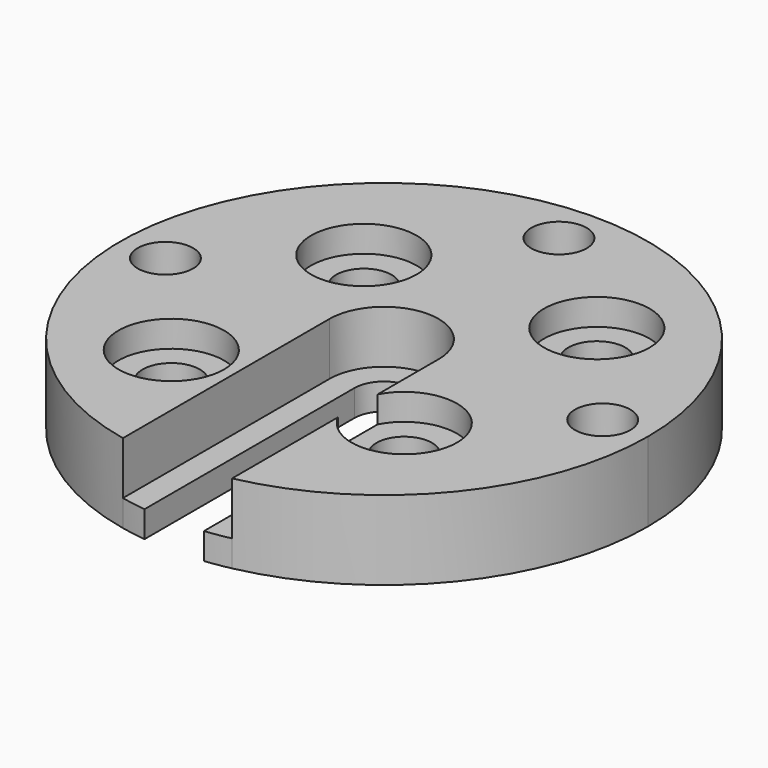
from build123d import *

# Parameters (mm, degrees)
F1_DEPTH = 1.5
F0_R     = 3
F0_R_2   = 1.575
F2_DEPTH = 4.5
F0_R_3   = 1.625
F3_DEPTH = 3


# Not quite as in the source:
# - a feature names something its author has since deleted; it is built from what else it names


with BuildPart() as f1:
    # F0 (on Top) → F1 (new body)
    with BuildSketch(Plane.XY):
        with BuildLine():
            Line((-1.685, -4.7075232341), (-1.685, -2.6020712903))
            ThreePointArc((-1.685, -2.6020712903), (-2.7233710728, -1.4809625248), (-3.1, 0))
            Line((-3.1, 0), (-3.1, -3.9230090492))
            ThreePointArc((-3.1, -3.9230090492), (-2.4244425909, -4.3728798432), (-1.685, -4.7075232341))
        make_face()
        with BuildLine():
            Line((-1.685, -14.905058705), (-1.685, -4.7075232341))
            ThreePointArc((-1.685, -4.7075232341), (-2.4244425909, -4.3728798432), (-3.1, -3.9230090492))
            Line((-3.1, -3.9230090492), (-3.1, -14.6761711628))
            ThreePointArc((-3.1, -14.6761711628), (-2.3952356099, -14.8075266798), (-1.685, -14.905058705))
        make_face()
        with BuildLine():
            ThreePointArc((3.1, -3.9230090492), (2.4244425909, -4.3728798432), (1.685, -4.7075232341))
            Line((1.685, -4.7075232341), (1.685, -14.905058705))
            ThreePointArc((1.685, -14.905058705), (2.3952356099, -14.8075266798), (3.1, -14.6761711628))
            Line((3.1, -14.6761711628), (3.1, -7.1604074647))
            ThreePointArc((3.1, -7.1604074647), (2.7452425971, -5.7452425971), (3.1, -4.3300777296))
            Line((3.1, -4.3300777296), (3.1, -3.9230090492))
        make_face()
        with BuildLine():
            ThreePointArc((-1.685, 0), (0, 1.685), (1.685, 0))
            Line((1.685, 0), (1.685, -2.6020712903))
            ThreePointArc((1.685, -2.6020712903), (2.7233710728, -1.4809625248), (3.1, 0))
            ThreePointArc((3.1, 0), (0, 3.1), (-3.1, 0))
            ThreePointArc((-3.1, 0), (-2.7233710728, -1.4809625248), (-1.685, -2.6020712903))
            Line((-1.685, -2.6020712903), (-1.685, 0))
        make_face()
        with BuildLine():
            ThreePointArc((-3.1, 0), (0, 3.1), (3.1, 0))
            Line((3.1, 0), (3.1, -3.9230090492))
            ThreePointArc((3.1, -3.9230090492), (4.5, -2.1794494718), (5, 0))
            ThreePointArc((5, 0), (-2.1794494718, 4.5), (-3.1, -3.9230090492))
            Line((-3.1, -3.9230090492), (-3.1, 0))
        make_face()
        with BuildLine():
            ThreePointArc((3.1, 0), (2.7233710728, -1.4809625248), (1.685, -2.6020712903))
            Line((1.685, -2.6020712903), (1.685, -4.7075232341))
            ThreePointArc((1.685, -4.7075232341), (2.4244425909, -4.3728798432), (3.1, -3.9230090492))
            Line((3.1, -3.9230090492), (3.1, 0))
        make_face()
        with BuildLine():
            Line((3.1, -7.1604074647), (3.1, -4.3300777296))
            ThreePointArc((3.1, -4.3300777296), (2.7452425971, -5.7452425971), (3.1, -7.1604074647))
        make_face()
    extrude(amount=F1_DEPTH)

    # F0 (on Top) → F2 (join)
    with BuildSketch(Plane.XY):
        with BuildLine():
            ThreePointArc((-3.1, 0), (0, 3.1), (3.1, 0))
            Line((3.1, 0), (3.1, -3.9230090492))
            ThreePointArc((3.1, -3.9230090492), (4.5, -2.1794494718), (5, 0))
            ThreePointArc((5, 0), (-2.1794494718, 4.5), (-3.1, -3.9230090492))
            Line((-3.1, -3.9230090492), (-3.1, 0))
        make_face()
        with BuildLine():
            ThreePointArc((5, 0), (4.5, -2.1794494718), (3.1, -3.9230090492))
            Line((3.1, -3.9230090492), (3.1, -4.3300777296))
            ThreePointArc((3.1, -4.3300777296), (6.4747191933, -2.8352831652), (8.7452425971, -5.7452425971))
            ThreePointArc((8.7452425971, -5.7452425971), (6.4747191933, -8.6552020291), (3.1, -7.1604074647))
            Line((3.1, -7.1604074647), (3.1, -14.6761711628))
            ThreePointArc((3.1, -14.6761711628), (11.6511801977, -9.4472218138), (15, 0))
            ThreePointArc((15, 0), (-9.4472218138, 11.6511801977), (-3.1, -14.6761711628))
            Line((-3.1, -14.6761711628), (-3.1, -3.9230090492))
            ThreePointArc((-3.1, -3.9230090492), (-2.1794494718, 4.5), (5, 0))
        make_face()
        with Locations((-6.7175144213, -6.7175144213)):
            Circle(F0_R, mode=Mode.SUBTRACT)
        with Locations((-12.425, 0)):
            Circle(F0_R_2, mode=Mode.SUBTRACT)
        with Locations((-5.7452425971, 5.7452425971)):
            Circle(F0_R, mode=Mode.SUBTRACT)
        with Locations((6.7175144213, 6.7175144213)):
            Circle(F0_R, mode=Mode.SUBTRACT)
        with Locations((12.425, 0)):
            Circle(F0_R_2, mode=Mode.SUBTRACT)
        with Locations((0, 12.425)):
            Circle(F0_R_2, mode=Mode.SUBTRACT)
    extrude(amount=F2_DEPTH)

    # F0 (on Top) → F3 (join)
    with BuildSketch(Plane.XY):
        with Locations((-5.7452425971, 5.7452425971)):
            Circle(F0_R)
        with Locations((-5.7452425971, 5.7452425971)):
            Circle(F0_R_2, mode=Mode.SUBTRACT)
        with Locations((6.7175144213, 6.7175144213)):
            Circle(F0_R)
        with Locations((6.7175144213, 6.7175144213)):
            Circle(F0_R_3, mode=Mode.SUBTRACT)
        with BuildLine():
            ThreePointArc((8.7452425971, -5.7452425971), (6.4747191933, -2.8352831652), (3.1, -4.3300777296))
            Line((3.1, -4.3300777296), (3.1, -7.1604074647))
            ThreePointArc((3.1, -7.1604074647), (6.4747191933, -8.6552020291), (8.7452425971, -5.7452425971))
        make_face()
        with Locations((5.7452425971, -5.7452425971)):
            Circle(F0_R_2, mode=Mode.SUBTRACT)
        with Locations((-6.7175144213, -6.7175144213)):
            Circle(F0_R)
        with Locations((-6.7175144213, -6.7175144213)):
            Circle(F0_R_3, mode=Mode.SUBTRACT)
    extrude(amount=F3_DEPTH)


solid = f1.part
